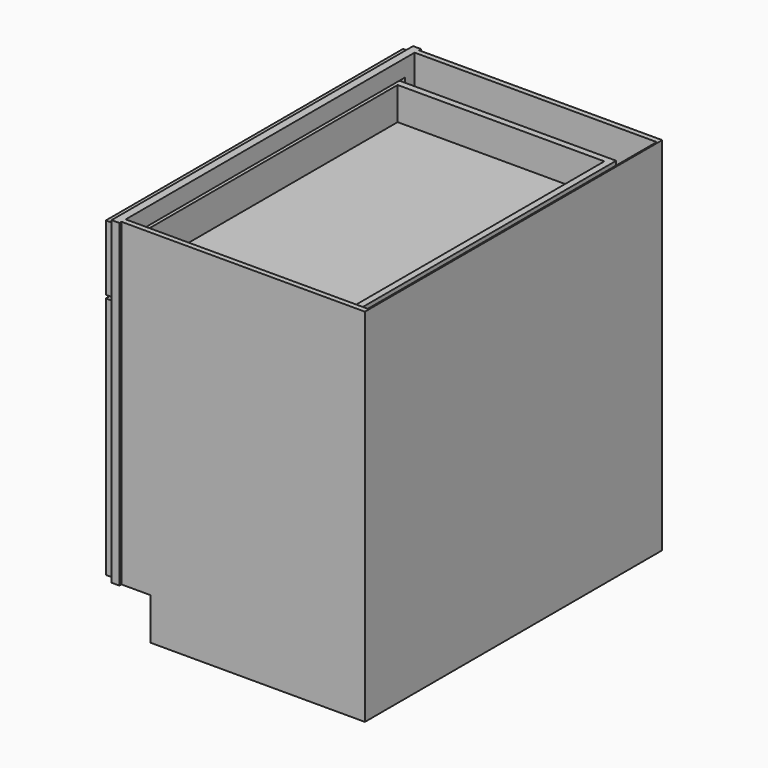
from build123d import *

# Parameters (mm, degrees)
F0_W          = 609.6
F0_H          = 876.3
F1_DEPTH      = 914.4
F2_W          = 88.9
F2_H          = 101.6
F3_DEPTH      = 914.401
F4_W          = 816.9639344262
F4_H          = 692.15
F5_DEPTH      = 19.05
F6_W          = 590.55
F6_H          = 6.35
F7_DEPTH      = 876.301
F8_W          = 587.375
F8_H          = 876.3
F9_DEPTH      = 733.425
F10_W         = 816.9639344262
F10_H         = 41.275
F11_DEPTH     = 19.05
F12_W         = 450.85
F12_H         = 590.5627
F12_W_2       = 336.55
F12_H_2       = 476.2627
F13_DEPTH     = 19.05
F14_W         = 6.35
F14_H         = 336.55
F15_DEPTH     = 476.2627
F16_SIZE      = 3.175
F17_W         = 901.7
F17_H         = 158.75
F17_W_2       = 787.4
F17_H_2       = 82.55
F18_DEPTH     = 19.05
F19_W         = 6.35
F19_H         = 787.4
F20_DEPTH     = 82.55
F21_SIZE      = 3.175
F22_W         = 504.825
F22_H         = 876.3
F23_DEPTH     = 101.6
F24_W         = 812.8
F24_H         = 95.25
F25_DEPTH     = 533.4
F26_T         = 15.875
F26_T3_DEPTH  = 37.249261314
F26_T5_DEPTH  = 37.249261314
F26_T7_DEPTH  = 37.249261314
F26_T9_DEPTH  = 37.249261314
F26_T11_DEPTH = 36.5125
F26_T13_DEPTH = 819.15
F26_T15_DEPTH = 114.3
F26_T17_DEPTH = 127
F26_T19_DEPTH = 844.55
F26_T21_DEPTH = 111.125
F26_T23_DEPTH = 36.5125


# Not quite as in the source:
# - a shell that OpenCascade refuses in one call is made with other operations: the cavity is built on its own and cut out


with BuildPart() as f1:
    # F0 (on Front) → F1 (new body)
    with BuildSketch(Plane.XZ):
        Rectangle(F0_W, F0_H)
    extrude(amount=-F1_DEPTH)

    # F2 (on face) → F3 (cut, through all)
    with BuildSketch(Plane.XZ):
        with Locations((-260.35, -387.35)):
            Rectangle(F2_W, F2_H)
    extrude(amount=-F3_DEPTH, mode=Mode.SUBTRACT)

    # F4 (on face) → F5 (cut)
    with BuildSketch(Plane(origin=(-304.8, 0, 0), x_dir=(0, -1, 0), z_dir=(-1, 0, 0))):
        with Locations((-457.2, 50.8)):
            Rectangle(F4_W, F4_H)
    extrude(amount=-F5_DEPTH, mode=Mode.SUBTRACT)

    # F6 (on face) → F7 (cut, through all)
    with BuildSketch(Plane.XY.offset(438.15)):
        with Locations((9.525, 911.225)):
            Rectangle(F6_W, F6_H)
        with Locations((9.525, 3.175)):
            Rectangle(F6_W, F6_H)
    extrude(amount=-F7_DEPTH, mode=Mode.SUBTRACT)

    # F8 (on face) → F9 (cut, through all)
    with BuildSketch(Plane.XY.offset(438.15)):
        with Locations((7.9375, 457.2)):
            Rectangle(F8_W, F8_H)
    extrude(amount=-F9_DEPTH, mode=Mode.SUBTRACT)

    # F10 (on face) → F11 (join, through all)
    with BuildSketch(Plane(origin=(-304.8, 0, 0), x_dir=(0, -1, 0), z_dir=(-1, 0, 0))):
        with Locations((-457.2, 265.1125)):
            Rectangle(F10_W, F10_H)
    extrude(amount=-F11_DEPTH)

    # F22 (on face) → F23 (cut)
    with BuildSketch(Plane(origin=(0, 0, -438.15), x_dir=(1, 0, 0), z_dir=(0, 0, -1))):
        with Locations((49.2125, -457.2)):
            Rectangle(F22_W, F22_H)
    extrude(amount=-F23_DEPTH, mode=Mode.SUBTRACT)


with BuildPart() as f13:
    # F12 (on face) → F13 (new body)
    with BuildSketch(Plane(origin=(-304.8, 0, 0), x_dir=(0, -1, 0), z_dir=(-1, 0, 0))):
        with Locations((-682.625, -33.33115)):
            Rectangle(F12_W, F12_H)
        with Locations((-682.625, -33.33115)):
            Rectangle(F12_W_2, F12_H_2, mode=Mode.SUBTRACT)
    extrude(amount=F13_DEPTH)

    # F14 (on face) → F15 (join, through all)
    with BuildSketch(Plane.XY.offset(-271.4625)):
        with Locations((-312.7375, 682.625)):
            Rectangle(F14_W, F14_H)
    extrude(amount=F15_DEPTH)

    # F16
    f16_edges = [f13.edges().sort_by_distance(p)[0] for p in [
        (-323.85, 850.9, -33.33115),
        (-323.85, 682.625, -271.4625),
        (-323.85, 514.35, -33.33115),
        (-323.85, 682.625, 204.8002),
    ]]
    chamfer(f16_edges, length=F16_SIZE)


with BuildPart() as f18:
    # F17 (on face) → F18 (new body)
    with BuildSketch(Plane(origin=(-304.8, 0, 0), x_dir=(0, -1, 0), z_dir=(-1, 0, 0))):
        with Locations((-457.2, 349.25)):
            Rectangle(F17_W, F17_H)
        with Locations((-457.2, 349.25)):
            Rectangle(F17_W_2, F17_H_2, mode=Mode.SUBTRACT)
    extrude(amount=F18_DEPTH)

    # F19 (on face) → F20 (join, through all)
    with BuildSketch(Plane.XY.offset(307.975)):
        with Locations((-312.7375, 457.2)):
            Rectangle(F19_W, F19_H)
    extrude(amount=F20_DEPTH)

    # F21
    f21_edges = [f18.edges().sort_by_distance(p)[0] for p in [
        (-323.85, 457.2, 307.975),
        (-323.85, 850.9, 349.25),
        (-323.85, 457.2, 390.525),
        (-323.85, 63.5, 349.25),
    ]]
    chamfer(f21_edges, length=F21_SIZE)

    # F24 (on face) → F25 (join)
    with BuildSketch(Plane.YZ.offset(-304.8)):
        with Locations((457.2, 339.725)):
            Rectangle(F24_W, F24_H)
    extrude(amount=F25_DEPTH)

    # F26: shell of thickness 15.875, made by hand


with BuildPart() as f26_core1:
    # F26_t2: copy of F18
    add(f18.part)

    # the walls: a layer under each face that stays
    f26_faces = [f26_core1.faces().sort_by_distance(p)[0] for p in [
        (-323.85, 757.7666666667, 296.3333333333),
        (-322.2625, 457.2, 306.3875),
        (-322.2625, 61.9125, 349.25),
        (-322.2625, 852.4875, 349.25),
        (-322.2625, 457.2, 392.1125),
        (-314.325, 457.2, 428.625),
        (-314.325, 908.05, 349.25),
        (-314.325, 457.2, 269.875),
        (-314.325, 6.35, 349.25),
        (-318.29375, 457.2, 307.975),
        (-318.29375, 63.5, 349.25),
        (-318.29375, 850.9, 349.25),
        (-318.29375, 457.2, 390.525),
        (-304.8, 757.7666666667, 402.1666666667),
        (-315.9125, 457.2, 349.25),
        (-38.1, 863.6, 339.725),
        (-38.1, 457.2, 292.1),
        (-38.1, 50.8, 339.725),
        (-307.18125, 63.5, 349.25),
        (-307.18125, 457.2, 390.525),
        (-307.18125, 850.9, 349.25),
        (-304.8, 457.2, 347.6625),
        (228.6, 457.2, 339.725),
        (-307.18125, 457.2, 307.975),
        (-309.5625, 457.2, 349.25),
    ]]
    thicken(f26_faces, amount=-F26_T, mode=Mode.SUBTRACT)

    # F26_s4 → F26_t3 (cut)
    with BuildSketch(Plane(origin=(4.5928978099, 4.5928978099, 4.5928978099), x_dir=(-0.7071067812, 0.7071067812, 0), z_dir=(0.5773502692, 0.5773502692, 0.5773502692))):
        Polygon((271.8908726623, 356.5892701441), (263.7152476623, 342.7036353262), (255.7777476623, 347.2863530879), (255.7777476623, 356.4517886113), align=None)
    extrude(amount=F26_T3_DEPTH, mode=Mode.SUBTRACT)

    # F26_s6 → F26_t5 (cut)
    with BuildSketch(Plane(origin=(-300.2071021901, 300.20710219, -300.2071021901), x_dir=(0.7071067812, 0.7071067812, 0), z_dir=(0.5773502692, -0.5773502692, 0.5773502692))):
        Polygon((374.6875680546, 729.8915069443), (382.8631930546, 716.0058721263), (390.8006930546, 720.588589888), (390.8006930546, 729.7540254114), align=None)
    extrude(amount=F26_T5_DEPTH, mode=Mode.SUBTRACT)

    # F26_s8 → F26_t7 (cut)
    with BuildSketch(Plane(origin=(-228.2404355234, -228.2404355234, 228.2404355234), x_dir=(-0.7071067812, 0.7071067812, 0), z_dir=(0.5773502692, 0.5773502692, -0.5773502692))):
        Polygon((271.8908726623, 213.7335916339), (255.7777476623, 213.8710731668), (255.7777476623, 223.0365086901), (263.7152476623, 227.6192264518), align=None)
    extrude(amount=F26_T7_DEPTH, mode=Mode.SUBTRACT)

    # F26_s10 → F26_t9 (cut)
    with BuildSketch(Plane(origin=(-533.0404355234, 533.0404355234, 533.0404355234), x_dir=(0.7071067812, 0.7071067812, 0), z_dir=(0.5773502692, -0.5773502692, -0.5773502692))):
        Polygon((374.6875680546, -159.5686451663), (390.8006930546, -159.4311636334), (390.8006930546, -150.26572811), (382.8631930546, -145.6830103483), align=None)
    extrude(amount=F26_T9_DEPTH, mode=Mode.SUBTRACT)

    # F26_s12 → F26_t11 (cut)
    with BuildSketch(Plane.YZ.offset(-336.55)):
        Polygon((850.74125, 308.13375), (850.9, 292.1), (866.775, 292.1), (866.775, 307.975), align=None)
        Polygon((63.65875, 308.13375), (63.5, 292.1), (47.625, 292.1), (47.625, 307.975), align=None)
        Polygon((63.65875, 390.36625), (47.625, 390.525), (47.625, 406.4), (63.5, 406.4), align=None)
        Polygon((850.74125, 390.36625), (866.775, 390.525), (866.775, 406.4), (850.9, 406.4), align=None)
    extrude(amount=F26_T11_DEPTH, mode=Mode.SUBTRACT)

    # F26_s14 → F26_t13 (cut)
    with BuildSketch(Plane.XZ.offset(-866.775)):
        Polygon((-316.07125, 308.13375), (-315.9125, 292.1), (-300.0375, 292.1), (-300.0375, 307.975), align=None)
        Polygon((-316.07125, 390.36625), (-315.9125, 406.4), (-300.0375, 406.4), (-300.0375, 390.525), align=None)
        Polygon((-309.40375, 390.36625), (-309.5625, 406.4), (-325.4375, 406.4), (-325.4375, 390.525), align=None)
        Polygon((-304.95875, 308.13375), (-288.925, 307.975), (-288.925, 292.1), (-304.8, 292.1), align=None)
        Polygon((-309.40375, 308.13375), (-309.5625, 292.1), (-325.4375, 292.1), (-325.4375, 307.975), align=None)
    extrude(amount=F26_T13_DEPTH, mode=Mode.SUBTRACT)

    # F26_s16 → F26_t15 (cut)
    with BuildSketch(Plane.XY.offset(292.1)):
        Polygon((-316.07125, 63.65875), (-315.9125, 47.625), (-300.0375, 47.625), (-300.0375, 63.5), align=None)
        Polygon((-316.07125, 850.74125), (-315.9125, 866.775), (-300.0375, 866.775), (-300.0375, 850.9), align=None)
        Polygon((-309.40375, 63.65875), (-309.5625, 47.625), (-325.4375, 47.625), (-325.4375, 63.5), align=None)
        Polygon((-309.40375, 850.74125), (-309.5625, 866.775), (-325.4375, 866.775), (-325.4375, 850.9), align=None)
    extrude(amount=F26_T15_DEPTH, mode=Mode.SUBTRACT)

    # F26_s18 → F26_t17 (cut)
    with BuildSketch(Plane.XY.offset(276.225)):
        Polygon((-304.64125, 863.75875), (-320.675, 863.6), (-320.675, 847.725), (-304.8, 847.725), align=None)
        Polygon((-304.64125, 50.64125), (-320.675, 50.8), (-320.675, 66.675), (-304.8, 66.675), align=None)
    extrude(amount=F26_T17_DEPTH, mode=Mode.SUBTRACT)

    # F26_s20 → F26_t19 (cut)
    with BuildSketch(Plane.XZ.offset(-879.475)):
        Polygon((-304.64125, 291.94125), (-320.675, 292.1), (-320.675, 307.975), (-304.8, 307.975), align=None)
    extrude(amount=F26_T19_DEPTH, mode=Mode.SUBTRACT)

    # F26_s22 → F26_t21 (cut)
    with BuildSketch(Plane.XY.offset(292.1)):
        Polygon((-304.95875, 63.65875), (-304.8, 47.625), (-288.925, 47.625), (-288.925, 63.5), align=None)
        Polygon((-304.95875, 850.74125), (-304.8, 866.775), (-288.925, 866.775), (-288.925, 850.9), align=None)
    extrude(amount=F26_T21_DEPTH, mode=Mode.SUBTRACT)

    # F26_s24 → F26_t23 (cut)
    with BuildSketch(Plane.YZ.offset(-325.4375)):
        Polygon((63.65875, 308.13375), (47.625, 307.975), (47.625, 292.1), (63.5, 292.1), align=None)
        Polygon((63.65875, 390.36625), (47.625, 390.525), (47.625, 406.4), (63.5, 406.4), align=None)
        Polygon((850.74125, 390.36625), (850.9, 406.4), (866.775, 406.4), (866.775, 390.525), align=None)
        Polygon((850.74125, 308.13375), (866.775, 307.975), (866.775, 292.1), (850.9, 292.1), align=None)
    extrude(amount=F26_T23_DEPTH, mode=Mode.SUBTRACT)


with BuildPart() as f18_1:
    add(f18.part)

    # what is left inside the walls is the cavity
    f26_cavity = [f26_core1.part.solids().sort_by_distance(p)[0] for p in [
        (45.508333, 457.2, 308.13375),
    ]]
    add(f26_cavity, mode=Mode.SUBTRACT)


with BuildPart() as f27_1:
    # F27: instance of F13
    add(f13.part.mirror(Plane(origin=(-314.325, 457.2, -33.33115), x_dir=(1, 0, 0), z_dir=(0, -1, 0))))


solid = Compound([f1.part, f13.part, f18_1.part, f27_1.part])
